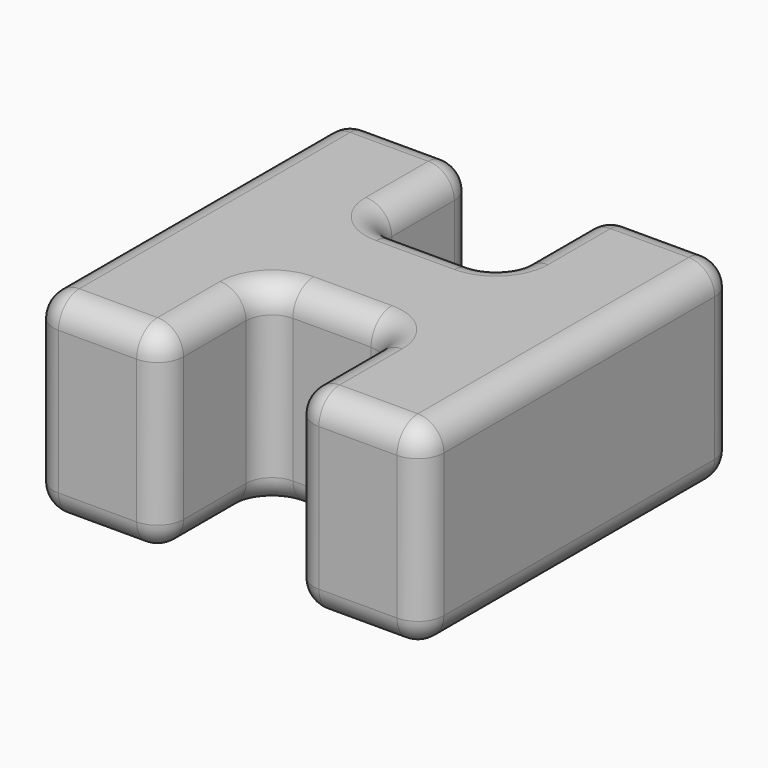
from build123d import *

# Parameters (mm, degrees)
F0_W     = 10
F0_H     = 10
F1_DEPTH = 15
F2_R     = 2


with BuildPart() as f1:
    # F0 (on Top) → F1 (new body)
    with BuildSketch(Plane.XY):
        Polygon((0, 30), (0, 0), (10, 0), (10, 10), (10, 20), (10, 30), align=None)
        with Locations((15, 15)):
            Rectangle(F0_W, F0_H)
        Polygon((20, 20), (20, 10), (20, 0), (30, 0), (30, 30), (20, 30), align=None)
    extrude(amount=F1_DEPTH)

    # F2
    f2_edges = [f1.edges().sort_by_distance(p)[0] for p in [
        (0, 30, 7.5),
        (20, 30, 7.5),
        (0, 0, 7.5),
        (10, 0, 7.5),
        (5, 0, 0),
        (5, 0, 15),
        (20, 0, 7.5),
        (30, 0, 7.5),
        (25, 0, 0),
        (25, 0, 15),
        (10, 20, 7.5),
        (10, 30, 7.5),
        (10, 25, 0),
        (10, 25, 15),
        (20, 20, 7.5),
        (20, 25, 0),
        (20, 25, 15),
        (30, 30, 7.5),
        (25, 30, 0),
        (25, 30, 15),
        (30, 15, 15),
        (10, 10, 7.5),
        (10, 5, 0),
        (10, 5, 15),
        (5, 30, 0),
        (5, 30, 15),
        (15, 20, 15),
        (20, 10, 7.5),
        (15, 10, 0),
        (15, 10, 15),
        (20, 5, 15),
        (0, 15, 0),
        (0, 15, 15),
        (30, 15, 0),
        (20, 5, 0),
        (15, 20, 0),
    ]]
    fillet(f2_edges, radius=F2_R)


solid = f1.part
